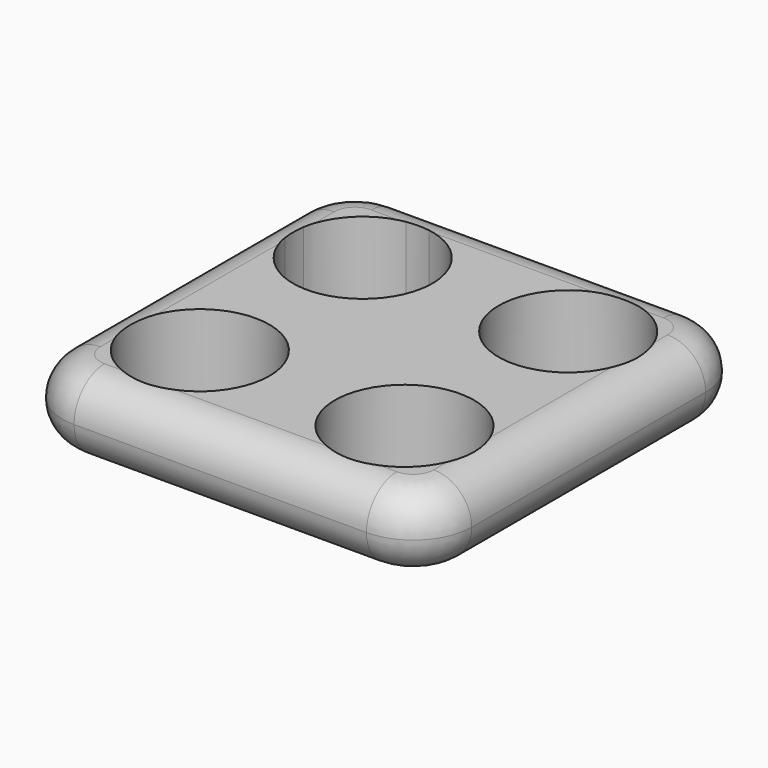
from build123d import *

# Parameters (mm, degrees)
F0_R         = 15.113
F1_DEPTH     = 16.51
F2_DEPTH     = 1.905
F3_T1_DEPTH  = 63.5
F3_T3_DEPTH  = 63.5
F3_T6_ANGLE  = 90
F3_T8_ANGLE  = 90
F3_T10_ANGLE = 90
F3_T12_ANGLE = 90
F3_T14_ANGLE = 90
F3_T16_ANGLE = 90
F3_T18_ANGLE = 90
F3_T20_ANGLE = 90


# Not quite as in the source:
# - a fillet or chamfer that OpenCascade refuses, or shapes differently, is made with other operations: its cross-section is extruded or revolved along the edge and cut away or added


with BuildPart() as f1:
    # F0 (on Top) → F1 (new body)
    with BuildSketch(Plane.XY):
        with BuildLine():
            Line((31.75, 44.45), (-31.75, 44.45))
            ThreePointArc((-31.75, 44.45), (-40.7302561211, 40.7302561211), (-44.45, 31.75))
            Line((-44.45, 31.75), (-44.45, -31.75))
            ThreePointArc((-44.45, -31.75), (-40.7302561211, -40.7302561211), (-31.75, -44.45))
            Line((-31.75, -44.45), (31.75, -44.45))
            ThreePointArc((31.75, -44.45), (40.7302561211, -40.7302561211), (44.45, -31.75))
            Line((44.45, -31.75), (44.45, 31.75))
            ThreePointArc((44.45, 31.75), (40.7302561211, 40.7302561211), (31.75, 44.45))
        make_face()
        with Locations((-22.225, -22.225)):
            Circle(F0_R, mode=Mode.SUBTRACT)
        with Locations((22.225, -22.225)):
            Circle(F0_R, mode=Mode.SUBTRACT)
        with BuildLine():
            ThreePointArc((-6.9787090866, 24.098385063), (-6.8187195919, 22.8373692451), (-6.7652637085, 21.5673692451))
            ThreePointArc((-6.7652637085, 21.5673692451), (-6.8187195919, 20.2973692451), (-6.9787090866, 19.0363534272))
            ThreePointArc((-6.9787090866, 19.0363534272), (-11.1917589244, 10.880864461), (-19.3472478905, 6.6678146232))
            ThreePointArc((-19.3472478905, 6.6678146232), (-21.8782637085, 6.4543692451), (-24.4092795264, 6.6678146232))
            ThreePointArc((-24.4092795264, 6.6678146232), (-32.5647684925, 10.880864461), (-36.7778183303, 19.0363534272))
            ThreePointArc((-36.7778183303, 19.0363534272), (-36.9912637085, 21.5673692451), (-36.7778183303, 24.098385063))
            ThreePointArc((-36.7778183303, 24.098385063), (-32.5647684925, 32.2538740292), (-24.4092795264, 36.4669238669))
            ThreePointArc((-24.4092795264, 36.4669238669), (-21.8782637085, 36.6803692451), (-19.3472478905, 36.4669238669))
            ThreePointArc((-19.3472478905, 36.4669238669), (-11.1917589244, 32.2538740292), (-6.9787090866, 24.098385063))
        make_face(mode=Mode.SUBTRACT)
        with Locations((22.225, 22.225)):
            Circle(F0_R, mode=Mode.SUBTRACT)
    extrude(amount=F1_DEPTH)

    # F0 (on Top) → F2 (join)
    with BuildSketch(Plane.XY):
        with BuildLine():
            ThreePointArc((-6.9787090866, 19.0363534272), (-6.8187195919, 20.2973692451), (-6.7652637085, 21.5673692451))
            ThreePointArc((-6.7652637085, 21.5673692451), (-6.8187195919, 22.8373692451), (-6.9787090866, 24.098385063))
            Line((-6.9787090866, 24.098385063), (-19.3472478905, 23.9739259511))
            ThreePointArc((-19.3472478905, 23.9739259511), (-18.6350300602, 22.8631283867), (-18.3857637085, 21.5673692451))
            ThreePointArc((-18.3857637085, 21.5673692451), (-18.668711127, 20.1902968152), (-19.4717070024, 19.0363534272))
            Line((-19.4717070024, 19.0363534272), (-6.9787090866, 19.0363534272))
        make_face()
        with BuildLine():
            Line((-19.3472478905, 23.9739259511), (-19.3472478905, 36.4669238669))
            ThreePointArc((-19.3472478905, 36.4669238669), (-21.8782637085, 36.6803692451), (-24.4092795264, 36.4669238669))
            Line((-24.4092795264, 36.4669238669), (-24.4092795264, 23.9739259511))
            ThreePointArc((-24.4092795264, 23.9739259511), (-21.8782637085, 25.0598692451), (-19.3472478905, 23.9739259511))
        make_face()
        with BuildLine():
            ThreePointArc((-18.3857637085, 21.5673692451), (-18.6350300602, 22.8631283867), (-19.3472478905, 23.9739259511))
            ThreePointArc((-19.3472478905, 23.9739259511), (-21.8782637085, 25.0598692451), (-24.4092795264, 23.9739259511))
            ThreePointArc((-24.4092795264, 23.9739259511), (-25.3707637085, 21.5673692451), (-24.4092795264, 19.160812539))
            ThreePointArc((-24.4092795264, 19.160812539), (-21.9662695904, 18.0759782308), (-19.4717070024, 19.0363534272))
            ThreePointArc((-19.4717070024, 19.0363534272), (-18.668711127, 20.1902968152), (-18.3857637085, 21.5673692451))
        make_face()
        with BuildLine():
            ThreePointArc((-24.4092795264, 19.160812539), (-25.3707637085, 21.5673692451), (-24.4092795264, 23.9739259511))
            Line((-24.4092795264, 23.9739259511), (-36.7778183303, 24.098385063))
            ThreePointArc((-36.7778183303, 24.098385063), (-36.9912637085, 21.5673692451), (-36.7778183303, 19.0363534272))
            Line((-36.7778183303, 19.0363534272), (-24.4092795264, 19.160812539))
        make_face()
        with BuildLine():
            ThreePointArc((-24.4092795264, 6.6678146232), (-21.8782637085, 6.4543692451), (-19.3472478905, 6.6678146232))
            Line((-19.3472478905, 6.6678146232), (-19.4717070024, 19.0363534272))
            ThreePointArc((-19.4717070024, 19.0363534272), (-21.9662695904, 18.0759782308), (-24.4092795264, 19.160812539))
            Line((-24.4092795264, 19.160812539), (-24.4092795264, 6.6678146232))
        make_face()
    extrude(amount=F2_DEPTH)

    # F3: fillet of radius 8.255 on 3 edges, made by hand

    # F3_s2 → F3_t1 (cut)
    with BuildSketch(Plane.XZ.offset(-31.75)):
        with BuildLine():
            ThreePointArc((-36.195, 16.51), (-42.0321664787, 14.0921664787), (-44.45, 8.255))
            Line((-44.45, 8.255), (-44.45, 16.51))
            Line((-44.45, 16.51), (-36.195, 16.51))
        make_face()
        with BuildLine():
            ThreePointArc((36.195, 0), (42.0321664787, 2.4178335213), (44.45, 8.255))
            Line((44.45, 8.255), (44.45, 0))
            Line((44.45, 0), (36.195, 0))
        make_face()
        with BuildLine():
            ThreePointArc((-36.195, 0), (-42.0321664787, 2.4178335213), (-44.45, 8.255))
            Line((-44.45, 8.255), (-44.45, 0))
            Line((-44.45, 0), (-36.195, 0))
        make_face()
        with BuildLine():
            ThreePointArc((36.195, 16.51), (42.0321664787, 14.0921664787), (44.45, 8.255))
            Line((44.45, 8.255), (44.45, 16.51))
            Line((44.45, 16.51), (36.195, 16.51))
        make_face()
    extrude(amount=F3_T1_DEPTH, mode=Mode.SUBTRACT)

    # F3_s4 → F3_t3 (cut)
    with BuildSketch(Plane.YZ.offset(-31.75)):
        with BuildLine():
            ThreePointArc((-36.195, 0), (-42.0321664787, 2.4178335213), (-44.45, 8.255))
            Line((-44.45, 8.255), (-44.45, 0))
            Line((-44.45, 0), (-36.195, 0))
        make_face()
        with BuildLine():
            ThreePointArc((44.45, 8.255), (42.0321664787, 2.4178335213), (36.195, 0))
            Line((36.195, 0), (44.45, 0))
            Line((44.45, 0), (44.45, 8.255))
        make_face()
        with BuildLine():
            ThreePointArc((-36.195, 16.51), (-42.0321664787, 14.0921664787), (-44.45, 8.255))
            Line((-44.45, 8.255), (-44.45, 16.51))
            Line((-44.45, 16.51), (-36.195, 16.51))
        make_face()
        with BuildLine():
            ThreePointArc((44.45, 8.255), (42.0321664787, 14.0921664787), (36.195, 16.51))
            Line((36.195, 16.51), (44.45, 16.51))
            Line((44.45, 16.51), (44.45, 8.255))
        make_face()
    extrude(amount=F3_T3_DEPTH, mode=Mode.SUBTRACT)

    # F3_s5 → F3_t6 (revolve, cut)
    with BuildSketch(Plane.YZ.offset(-31.75)):
        with BuildLine():
            ThreePointArc((44.45, 8.255), (42.0321664787, 14.0921664787), (36.195, 16.51))
            Line((36.195, 16.51), (44.45, 16.51))
            Line((44.45, 16.51), (44.45, 8.255))
        make_face()
    revolve(axis=Axis((-31.75, 31.75, 16.51), (0, 0, 1)), revolution_arc=F3_T6_ANGLE, mode=Mode.SUBTRACT)

    # F3_s7 → F3_t8 (revolve, cut)
    with BuildSketch(Plane.XZ.offset(31.75)):
        with BuildLine():
            ThreePointArc((-36.195, 0), (-42.0321664787, 2.4178335213), (-44.45, 8.255))
            Line((-44.45, 8.255), (-44.45, 0))
            Line((-44.45, 0), (-36.195, 0))
        make_face()
    revolve(axis=Axis((-31.75, -31.75, 0), (0, 0, 1)), revolution_arc=F3_T8_ANGLE, mode=Mode.SUBTRACT)

    # F3_s9 → F3_t10 (revolve, cut)
    with BuildSketch(Plane.YZ.offset(31.75)):
        with BuildLine():
            ThreePointArc((-36.195, 0), (-42.0321664787, 2.4178335213), (-44.45, 8.255))
            Line((-44.45, 8.255), (-44.45, 0))
            Line((-44.45, 0), (-36.195, 0))
        make_face()
    revolve(axis=Axis((31.75, -31.75, 0), (0, 0, 1)), revolution_arc=F3_T10_ANGLE, mode=Mode.SUBTRACT)

    # F3_s11 → F3_t12 (revolve, cut)
    with BuildSketch(Plane.XZ.offset(-31.75)):
        with BuildLine():
            ThreePointArc((44.45, 8.255), (42.0321664787, 2.4178335213), (36.195, 0))
            Line((36.195, 0), (44.45, 0))
            Line((44.45, 0), (44.45, 8.255))
        make_face()
    revolve(axis=Axis((31.75, 31.75, 0), (0, 0, 1)), revolution_arc=F3_T12_ANGLE, mode=Mode.SUBTRACT)

    # F3_s13 → F3_t14 (revolve, cut)
    with BuildSketch(Plane.YZ.offset(-31.75)):
        with BuildLine():
            ThreePointArc((44.45, 8.255), (42.0321664787, 2.4178335213), (36.195, 0))
            Line((36.195, 0), (44.45, 0))
            Line((44.45, 0), (44.45, 8.255))
        make_face()
    revolve(axis=Axis((-31.75, 31.75, 0), (0, 0, 1)), revolution_arc=F3_T14_ANGLE, mode=Mode.SUBTRACT)

    # F3_s15 → F3_t16 (revolve, cut)
    with BuildSketch(Plane.XZ.offset(31.75)):
        with BuildLine():
            ThreePointArc((-36.195, 16.51), (-42.0321664787, 14.0921664787), (-44.45, 8.255))
            Line((-44.45, 8.255), (-44.45, 16.51))
            Line((-44.45, 16.51), (-36.195, 16.51))
        make_face()
    revolve(axis=Axis((-31.75, -31.75, 16.51), (0, 0, 1)), revolution_arc=F3_T16_ANGLE, mode=Mode.SUBTRACT)

    # F3_s17 → F3_t18 (revolve, cut)
    with BuildSketch(Plane.YZ.offset(31.75)):
        with BuildLine():
            ThreePointArc((-36.195, 16.51), (-42.0321664787, 14.0921664787), (-44.45, 8.255))
            Line((-44.45, 8.255), (-44.45, 16.51))
            Line((-44.45, 16.51), (-36.195, 16.51))
        make_face()
    revolve(axis=Axis((31.75, -31.75, 16.51), (0, 0, 1)), revolution_arc=F3_T18_ANGLE, mode=Mode.SUBTRACT)

    # F3_s19 → F3_t20 (revolve, cut)
    with BuildSketch(Plane.XZ.offset(-31.75)):
        with BuildLine():
            ThreePointArc((44.45, 8.255), (42.0321664787, 14.0921664787), (36.195, 16.51))
            Line((36.195, 16.51), (44.45, 16.51))
            Line((44.45, 16.51), (44.45, 8.255))
        make_face()
    revolve(axis=Axis((31.75, 31.75, 16.51), (0, 0, 1)), revolution_arc=F3_T20_ANGLE, mode=Mode.SUBTRACT)


solid = f1.part
